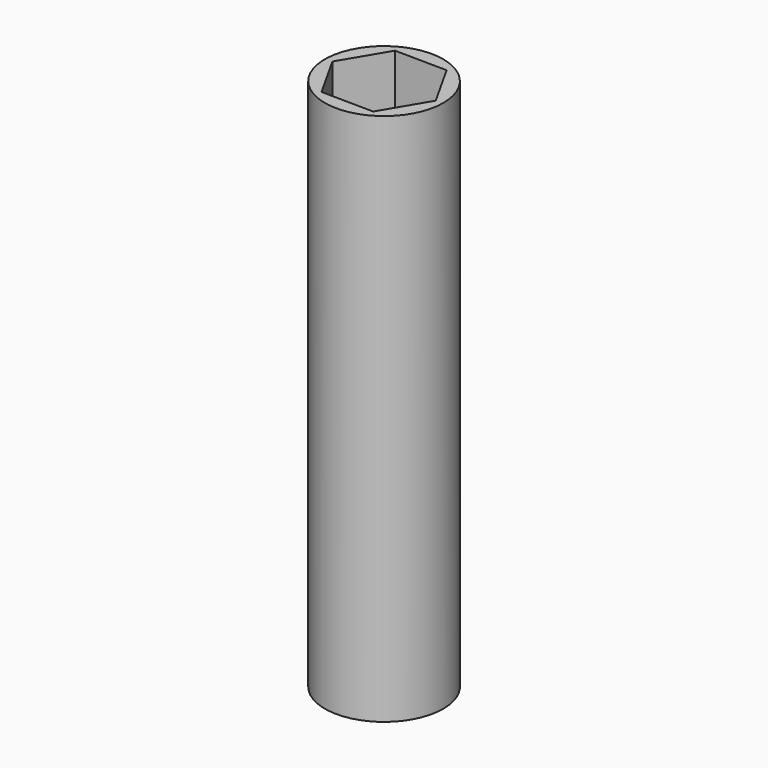
from build123d import *

# Parameters (mm, degrees)
F0_R     = 7.493
F0_R_2   = 5.08
F0_R_3   = 3.429
F1_DEPTH = 67.4878
F2_R     = 5.08
F2_R_2   = 3.429
F3_DEPTH = 5.08
F4_SIZE  = 1.65099
F5_R     = 3.429
F6_DEPTH = 7.62


# Not quite as in the source:
# - a fillet or chamfer is up to 0.001 mm smaller than in the source, because OpenCascade refuses the exact size


with BuildPart() as f1:
    # F0 (on Top) → F1 (new body)
    with BuildSketch(Plane.XY):
        Circle(F0_R)
        Circle(F0_R_2, mode=Mode.SUBTRACT)
        Circle(F0_R_2)
        Circle(F0_R_3, mode=Mode.SUBTRACT)
    extrude(amount=F1_DEPTH)

    # F2 (on face) → F3 (cut)
    with BuildSketch(Plane(origin=(0, 0, 0), x_dir=(1, 0, 0), z_dir=(0, 0, -1))):
        Circle(F2_R)
        Circle(F2_R_2, mode=Mode.SUBTRACT)
    extrude(amount=-F3_DEPTH, mode=Mode.SUBTRACT)

    # F4 (size 1.651 in the source; OpenCascade refuses exactly that, so slightly less here)
    f4_edges = [f1.edges().sort_by_distance(p)[0] for p in [
        (-3.429, 0, 5.08),
    ]]
    chamfer(f4_edges, length=F4_SIZE)

    # F5 (on face) → F6 (cut)
    with BuildSketch(Plane.XY.offset(67.4878)):
        Polygon((6.6034672536, -0.0838822432), (3.3743777803, 5.6768292731), (-3.2290894733, 5.7607115163), (-6.6034672536, 0.0838822432), (-3.3743777803, -5.6768292731), (3.2290894733, -5.7607115163), align=None)
        Circle(F5_R, mode=Mode.SUBTRACT)
        Circle(F5_R)
    extrude(amount=-F6_DEPTH, mode=Mode.SUBTRACT)


solid = f1.part
